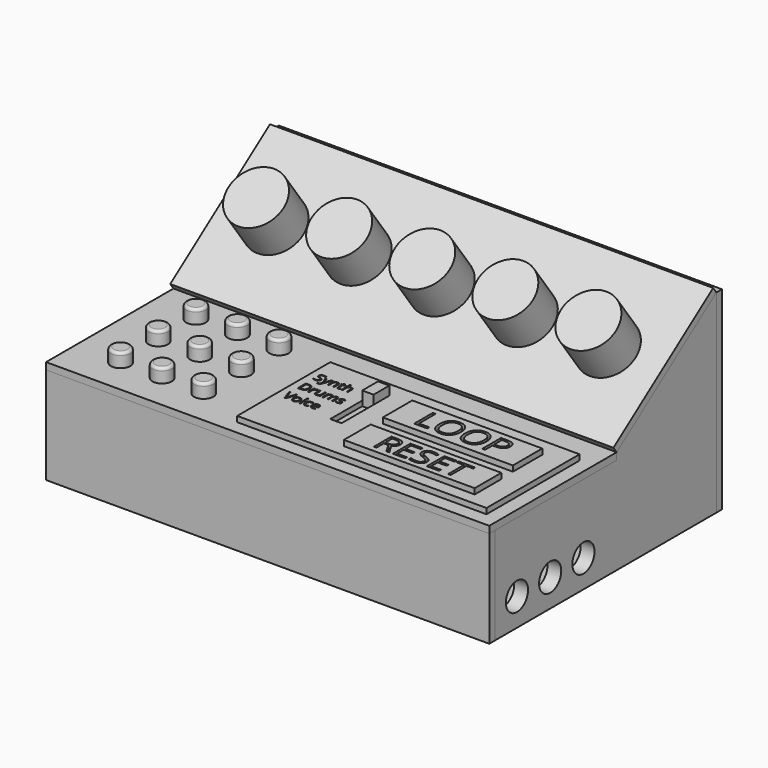
from build123d import *

# Parameters (mm, degrees)
F0_W          = 203.2
F0_H          = 127
F1_DEPTH      = 6.35
F2_W          = 63.5
F2_H          = 38.1
F3_DEPTH      = 6.35
F5_DEPTH      = 6.35
F6_W          = 203.2
F6_H          = 70.496440513
F7_DEPTH      = 3.175
F9_DEPTH      = 3.175
F10_W         = 203.2
F10_H         = 44.45
F11_DEPTH     = 3.175
F12_W         = 203.2
F12_H         = 88.9
F13_DEPTH     = 3.175
F14_R         = 12.7
F15_DEPTH     = 19.05
F16_R         = 6.35
F17_DEPTH     = 25.4
F18_R         = 26.0740110677
F19_DEPTH     = 6.35
F20_R         = 6.34999
F21_W         = 114.3
F21_H         = 53.34
F22_DEPTH     = 2.54
F23_TEXT_SIZE = 6.4763732048
F24_DEPTH     = 1.27
F25_W         = 5.1960833371
F25_H         = 27.3660402745
F26_DEPTH     = 2.286
F27_W         = 5.1960833371
F27_H         = 9.0065440163
F28_DEPTH     = 6.35
F29_W         = 59.6115607768
F29_H         = 16.8355405331
F30_DEPTH     = 2.54
F29_W_2       = 59.9551443011
F29_H_2       = 15.2894221246
F32_R         = 4.445
F33_DEPTH     = 6.35
F34_R         = 1.27
F34_2_R       = 1.27
F34_3_R       = 1.27
F34_4_R       = 1.27
F34_5_R       = 1.27
F34_6_R       = 1.27
F34_7_R       = 1.27
F34_8_R       = 1.27
F34_9_R       = 1.27


# Not quite as in the source:
# - a fillet or chamfer is up to 0.001 mm smaller than in the source, because OpenCascade refuses the exact size
# - Text() gives the source's letters only with a copy of the font that has no kerning and outlines rounded to 1/6400 em; it was checked with that copy


with BuildPart() as f1:
    # F0 (on Top) → F1 (new body)
    with BuildSketch(Plane.XY):
        Rectangle(F0_W, F0_H)
    extrude(amount=F1_DEPTH)

    # F2 (on face) → F3 (join)
    with BuildSketch(Plane(origin=(-101.6, 0, 0), x_dir=(0, -1, 0), z_dir=(-1, 0, 0))):
        Polygon((-63.5, 88.9), (-63.5, 6.35), (0, 6.35), (0, 44.45), (-6.35, 44.45), (-6.35, 47.625), align=None)
        with Locations((31.75, 25.4)):
            Rectangle(F2_W, F2_H)
    extrude(amount=-F3_DEPTH)

    # F4 (on face) → F5 (join)
    with BuildSketch(Plane.YZ.offset(101.6)):
        Polygon((-63.5, 44.45), (-63.5, 6.35), (63.5, 6.35), (63.5, 88.9), (6.35, 47.625), (6.35, 44.45), align=None)
    extrude(amount=-F5_DEPTH)

    # F16 (on face) → F17 (cut)
    with BuildSketch(Plane.YZ.offset(101.6)):
        with Locations((-50.8, 12.7)):
            Circle(F16_R)
        with Locations((-31.75, 12.7)):
            Circle(F16_R)
        with Locations((-12.7, 12.7)):
            Circle(F16_R)
    extrude(amount=-F17_DEPTH, mode=Mode.SUBTRACT)


with BuildPart() as f7:
    # F6 (on face) → F7 (new body)
    with BuildSketch(Plane(origin=(0, -20.4281947262, 28.2851926978), x_dir=(1, 0, 0), z_dir=(0, -0.5854905538, 0.8106792284))):
        with Locations((0, 68.2800209837)):
            Rectangle(F6_W, F6_H)
    extrude(amount=F7_DEPTH)


with BuildPart() as f9:
    # F8 (on face) → F9 (new body)
    with BuildSketch(Plane.XY.offset(44.45)):
        Polygon((101.6, 6.35), (-101.6, 6.35), (-101.6, -66.675), (101.6, -66.675), (101.6, -63.5), align=None)
    extrude(amount=F9_DEPTH)

    # F21 (on face) → F22 (join)
    with BuildSketch(Plane.XY.offset(47.625)):
        with Locations((38.1, -33.655)):
            Rectangle(F21_W, F21_H)
    extrude(amount=F22_DEPTH)

    # F23 (on face) → F24 (cut)
    with BuildSketch(Plane.XY.offset(50.165)):
        with Locations((-16.209024936, -21.1453055963)):
            Text('Synth', F23_TEXT_SIZE, font='Open Sans', text_align=(TextAlign.LEFT, TextAlign.BOTTOM))
        with Locations((-16.209024936, -29.9531731548)):
            Text('Drums', F23_TEXT_SIZE, font='Open Sans', text_align=(TextAlign.LEFT, TextAlign.BOTTOM))
        with Locations((-16.209024936, -38.7610407132)):
            Text('Voice', F23_TEXT_SIZE, font='Open Sans', text_align=(TextAlign.LEFT, TextAlign.BOTTOM))
    extrude(amount=-F24_DEPTH, mode=Mode.SUBTRACT)

    # F25 (on face) → F26 (cut)
    with BuildSketch(Plane.XY.offset(50.165)):
        with Locations((11.0760945827, -27.7290083468)):
            Rectangle(F25_W, F25_H)
    extrude(amount=-F26_DEPTH, mode=Mode.SUBTRACT)


with BuildPart() as f11:
    # F10 (on face) → F11 (new body)
    with BuildSketch(Plane.XZ.offset(63.5)):
        with Locations((0, 22.225)):
            Rectangle(F10_W, F10_H)
    extrude(amount=F11_DEPTH)


with BuildPart() as f13:
    # F12 (on face) → F13 (new body)
    with BuildSketch(Plane(origin=(0, 63.5, 0), x_dir=(-1, 0, 0), z_dir=(0, 1, 0))):
        with Locations((0, 44.45)):
            Rectangle(F12_W, F12_H)
    extrude(amount=F13_DEPTH)


with BuildPart() as f15:
    # F14 (on face) → F15 (new body)
    with BuildSketch(Plane(origin=(0, -22.2871272346, 30.8590992479), x_dir=(1, 0, 0), z_dir=(0, -0.5854905538, 0.8106792284))):
        with Locations((76.2, 68.2800209837)):
            Circle(F14_R)
    extrude(amount=F15_DEPTH)


with BuildPart() as f15b:
    # F14 (on face) → F15, piece 2 (new body)
    with BuildSketch(Plane(origin=(0, -22.2871272346, 30.8590992479), x_dir=(1, 0, 0), z_dir=(0, -0.5854905538, 0.8106792284))):
        with Locations((38.1, 68.2800209837)):
            Circle(F14_R)
    extrude(amount=F15_DEPTH)


with BuildPart() as f15c:
    # F14 (on face) → F15, piece 3 (new body)
    with BuildSketch(Plane(origin=(0, -22.2871272346, 30.8590992479), x_dir=(1, 0, 0), z_dir=(0, -0.5854905538, 0.8106792284))):
        with Locations((0, 68.2800209837)):
            Circle(F14_R)
    extrude(amount=F15_DEPTH)


with BuildPart() as f15d:
    # F14 (on face) → F15, piece 4 (new body)
    with BuildSketch(Plane(origin=(0, -22.2871272346, 30.8590992479), x_dir=(1, 0, 0), z_dir=(0, -0.5854905538, 0.8106792284))):
        with Locations((-38.1, 68.2800209837)):
            Circle(F14_R)
    extrude(amount=F15_DEPTH)


with BuildPart() as f15e:
    # F14 (on face) → F15, piece 5 (new body)
    with BuildSketch(Plane(origin=(0, -22.2871272346, 30.8590992479), x_dir=(1, 0, 0), z_dir=(0, -0.5854905538, 0.8106792284))):
        with Locations((-76.2, 68.2800209837)):
            Circle(F14_R)
    extrude(amount=F15_DEPTH)


with BuildPart() as f19:
    # F18 (on face) → F19 (new body)
    with BuildSketch(Plane.XY.offset(47.625)):
        with Locations((-63.5, -34.925)):
            Circle(F18_R)
    extrude(amount=F19_DEPTH)

    # F20 (radius 6.35 in the source; OpenCascade refuses exactly that, so slightly less here)
    f20_edges = [f19.edges().sort_by_distance(p)[0] for p in [
        (-89.574011, -34.925, 53.975),
    ]]
    fillet(f20_edges, radius=F20_R)


with BuildPart() as f28:
    # F27 (on face) → F28 (new body)
    with BuildSketch(Plane.XY.offset(47.879)):
        with Locations((11.0760945827, -18.5492602177)):
            Rectangle(F27_W, F27_H)
    extrude(amount=F28_DEPTH)


with BuildPart() as f30:
    # F29 (on face) → F30 (new body)
    with BuildSketch(Plane.XY.offset(50.165)):
        with Locations((55.256693624, -24.043854326)):
            Rectangle(F29_W, F29_H)
        Polygon((43.2155371847, -29.1975922883), (37.2333763145, -29.1975922883), (37.2333763145, -18.4663425765), (38.4805405948, -18.4663425765), (38.4805405948, -28.0678634392), (43.2155371847, -28.0678634392), align=None, mode=Mode.SUBTRACT)
        with BuildLine():
            add(Edge.make_bspline(
                [(53.05192891, -19.7651784466), (54.3507647801, -21.2331213378), (54.3507647801, -23.8167008263)],
                knots=[0, 0, 0, 1, 1, 1], degree=2))
            add(Edge.make_bspline(
                [(54.3507647801, -23.8167008263), (54.3507647801, -26.3932341889), (53.0472314927, -27.8693975603)],
                knots=[0, 0, 0, 1, 1, 1], degree=2))
            add(Edge.make_bspline(
                [(53.0472314927, -27.8693975603), (51.7436982053, -29.3455609317), (49.4255227916, -29.3455609317)],
                knots=[0, 0, 0, 1, 1, 1], degree=2))
            add(Edge.make_bspline(
                [(49.4255227916, -29.3455609317), (47.055675788, -29.3455609317), (45.7674091067, -27.8952333552)],
                knots=[0, 0, 0, 1, 1, 1], degree=2))
            add(Edge.make_bspline(
                [(45.7674091067, -27.8952333552), (44.4791424254, -26.4449057787), (44.4791424254, -23.8026085745)],
                knots=[0, 0, 0, 1, 1, 1], degree=2))
            add(Edge.make_bspline(
                [(44.4791424254, -23.8026085745), (44.4791424254, -21.181449748), (45.7709321696, -19.7393426517)],
                knots=[0, 0, 0, 1, 1, 1], degree=2))
            add(Edge.make_bspline(
                [(45.7709321696, -19.7393426517), (47.0627219139, -18.2972355554), (49.4396150433, -18.2972355554)],
                knots=[0, 0, 0, 1, 1, 1], degree=2))
            add(Edge.make_bspline(
                [(49.4396150433, -18.2972355554), (51.7530930398, -18.2972355554), (53.05192891, -19.7651784466)],
                knots=[0, 0, 0, 1, 1, 1], degree=2))
        make_face(mode=Mode.SUBTRACT)
        with BuildLine():
            add(Edge.make_bspline(
                [(64.7578927015, -19.7651784466), (66.0567285716, -21.2331213378), (66.0567285716, -23.8167008263)],
                knots=[0, 0, 0, 1, 1, 1], degree=2))
            add(Edge.make_bspline(
                [(66.0567285716, -23.8167008263), (66.0567285716, -26.3932341889), (64.7531952842, -27.8693975603)],
                knots=[0, 0, 0, 1, 1, 1], degree=2))
            add(Edge.make_bspline(
                [(64.7531952842, -27.8693975603), (63.4496619969, -29.3455609317), (61.1314865831, -29.3455609317)],
                knots=[0, 0, 0, 1, 1, 1], degree=2))
            add(Edge.make_bspline(
                [(61.1314865831, -29.3455609317), (58.7616395795, -29.3455609317), (57.4733728982, -27.8952333552)],
                knots=[0, 0, 0, 1, 1, 1], degree=2))
            add(Edge.make_bspline(
                [(57.4733728982, -27.8952333552), (56.1851062169, -26.4449057787), (56.1851062169, -23.8026085745)],
                knots=[0, 0, 0, 1, 1, 1], degree=2))
            add(Edge.make_bspline(
                [(56.1851062169, -23.8026085745), (56.1851062169, -21.181449748), (57.4768959612, -19.7393426517)],
                knots=[0, 0, 0, 1, 1, 1], degree=2))
            add(Edge.make_bspline(
                [(57.4768959612, -19.7393426517), (58.7686857054, -18.2972355554), (61.1455788348, -18.2972355554)],
                knots=[0, 0, 0, 1, 1, 1], degree=2))
            add(Edge.make_bspline(
                [(61.1455788348, -18.2972355554), (63.4590568314, -18.2972355554), (64.7578927015, -19.7651784466)],
                knots=[0, 0, 0, 1, 1, 1], degree=2))
        make_face(mode=Mode.SUBTRACT)
        with BuildLine():
            add(Edge.make_bspline(
                [(71.2309336745, -18.4663425765), (75.251922842, -18.4663425765), (75.251922842, -21.5924737576)],
                knots=[0, 0, 0, 1, 1, 1], degree=2))
            add(Edge.make_bspline(
                [(75.251922842, -21.5924737576), (75.251922842, -23.2224775439), (74.1398093077, -24.0997202157)],
                knots=[0, 0, 0, 1, 1, 1], degree=2))
            add(Edge.make_bspline(
                [(74.1398093077, -24.0997202157), (73.0276957733, -24.9769628875), (70.9584834739, -24.9769628875)],
                knots=[0, 0, 0, 1, 1, 1], degree=2))
            Line((70.9584834739, -24.9769628875), (69.6948782331, -24.9769628875))
            Line((69.6948782331, -24.9769628875), (69.6948782331, -29.1975922883))
            Line((69.6948782331, -29.1975922883), (68.4477139528, -29.1975922883))
            Line((68.4477139528, -29.1975922883), (68.4477139528, -18.4663425765))
            Line((68.4477139528, -18.4663425765), (71.2309336745, -18.4663425765))
        make_face(mode=Mode.SUBTRACT)
    extrude(amount=F30_DEPTH)


with BuildPart() as f30b:
    # F29 (on face) → F30, piece 2 (new body)
    with BuildSketch(Plane.XY.offset(50.165)):
        with Locations((55.4284853861, -47.1497792751)):
            Rectangle(F29_W_2, F29_H_2)
        with BuildLine():
            Line((40.4061070812, -48.0384091174), (38.3077044907, -48.0384091174))
            Line((38.3077044907, -48.0384091174), (38.3077044907, -52.217617631))
            Line((38.3077044907, -52.217617631), (37.1397256903, -52.217617631))
            Line((37.1397256903, -52.217617631), (37.1397256903, -42.1677209476))
            Line((37.1397256903, -42.1677209476), (39.8958037258, -42.1677209476))
            add(Edge.make_bspline(
                [(39.8958037258, -42.1677209476), (41.7456533889, -42.1677209476), (42.6287861353, -42.8759868114)],
                knots=[0, 0, 0, 1, 1, 1], degree=2))
            add(Edge.make_bspline(
                [(42.6287861353, -42.8759868114), (43.5119188818, -43.5842526753), (43.5119188818, -45.0073831534)],
                knots=[0, 0, 0, 1, 1, 1], degree=2))
            add(Edge.make_bspline(
                [(43.5119188818, -45.0073831534), (43.5119188818, -47.0002057393), (41.4905017112, -47.7018728529)],
                knots=[0, 0, 0, 1, 1, 1], degree=2))
            Line((41.4905017112, -47.7018728529), (44.2201847456, -52.217617631))
            Line((44.2201847456, -52.217617631), (42.8388463527, -52.217617631))
            Line((42.8388463527, -52.217617631), (40.4061070812, -48.0384091174))
        make_face(mode=Mode.SUBTRACT)
        Polygon((51.4436167238, -51.1728155026), (51.4436167238, -52.217617631), (45.8412777322, -52.217617631), (45.8412777322, -42.1677209476), (51.4436167238, -42.1677209476), (51.4436167238, -43.2059243257), (47.0092565326, -43.2059243257), (47.0092565326, -46.443711132), (51.1752675456, -46.443711132), (51.1752675456, -47.4753157598), (47.0092565326, -47.4753157598), (47.0092565326, -51.1728155026), align=None, mode=Mode.SUBTRACT)
        with BuildLine():
            add(Edge.make_bspline(
                [(58.7462337054, -47.86684161), (59.340121231, -48.5135191379), (59.340121231, -49.5429241823)],
                knots=[0, 0, 0, 1, 1, 1], degree=2))
            add(Edge.make_bspline(
                [(59.340121231, -49.5429241823), (59.340121231, -50.8692729895), (58.3778034812, -51.6127321882)],
                knots=[0, 0, 0, 1, 1, 1], degree=2))
            add(Edge.make_bspline(
                [(58.3778034812, -51.6127321882), (57.4154857313, -52.3561913869), (55.7657981602, -52.3561913869)],
                knots=[0, 0, 0, 1, 1, 1], degree=2))
            add(Edge.make_bspline(
                [(55.7657981602, -52.3561913869), (53.9797364165, -52.3561913869), (53.016318875, -51.894278867)],
                knots=[0, 0, 0, 1, 1, 1], degree=2))
            Line((53.016318875, -51.894278867), (53.016318875, -50.7680921518))
            add(Edge.make_bspline(
                [(53.016318875, -50.7680921518), (53.6366014017, -51.0276429963), (54.3646635164, -51.1794142529)],
                knots=[0, 0, 0, 1, 1, 1], degree=2))
            add(Edge.make_bspline(
                [(54.3646635164, -51.1794142529), (55.0927256312, -51.3311855094), (55.8075902453, -51.3311855094)],
                knots=[0, 0, 0, 1, 1, 1], degree=2))
            add(Edge.make_bspline(
                [(55.8075902453, -51.3311855094), (56.9755690457, -51.3311855094), (57.5672569879, -50.8879694486)],
                knots=[0, 0, 0, 1, 1, 1], degree=2))
            add(Edge.make_bspline(
                [(57.5672569879, -50.8879694486), (58.1589449301, -50.4447533878), (58.1589449301, -49.6529033537)],
                knots=[0, 0, 0, 1, 1, 1], degree=2))
            add(Edge.make_bspline(
                [(58.1589449301, -49.6529033537), (58.1589449301, -49.1316020812), (57.9488847127, -48.7983651918)],
                knots=[0, 0, 0, 1, 1, 1], degree=2))
            add(Edge.make_bspline(
                [(57.9488847127, -48.7983651918), (57.7388244953, -48.4651283025), (57.2472175991, -48.1824818319)],
                knots=[0, 0, 0, 1, 1, 1], degree=2))
            add(Edge.make_bspline(
                [(57.2472175991, -48.1824818319), (56.7556107029, -47.8998353614), (55.7526006596, -47.5435028461)],
                knots=[0, 0, 0, 1, 1, 1], degree=2))
            add(Edge.make_bspline(
                [(55.7526006596, -47.5435028461), (54.3514660159, -47.0419978244), (53.7498799483, -46.3546280031)],
                knots=[0, 0, 0, 1, 1, 1], degree=2))
            add(Edge.make_bspline(
                [(53.7498799483, -46.3546280031), (53.1482938806, -45.6672581818), (53.1482938806, -44.5608677174)],
                knots=[0, 0, 0, 1, 1, 1], degree=2))
            add(Edge.make_bspline(
                [(53.1482938806, -44.5608677174), (53.1482938806, -43.3994876674), (54.0204287099, -42.712117846)],
                knots=[0, 0, 0, 1, 1, 1], degree=2))
            add(Edge.make_bspline(
                [(54.0204287099, -42.712117846), (54.8925635392, -42.0247480247), (56.3310911012, -42.0247480247)],
                knots=[0, 0, 0, 1, 1, 1], degree=2))
            add(Edge.make_bspline(
                [(56.3310911012, -42.0247480247), (57.8290074158, -42.0247480247), (59.0871691367, -42.5746438818)],
                knots=[0, 0, 0, 1, 1, 1], degree=2))
            Line((59.0871691367, -42.5746438818), (58.7220382877, -43.5908514256))
            add(Edge.make_bspline(
                [(58.7220382877, -43.5908514256), (57.4770740673, -43.0695501531), (56.3024965167, -43.0695501531)],
                knots=[0, 0, 0, 1, 1, 1], degree=2))
            add(Edge.make_bspline(
                [(56.3024965167, -43.0695501531), (55.37427231, -43.0695501531), (54.8518712458, -43.4676747536)],
                knots=[0, 0, 0, 1, 1, 1], degree=2))
            add(Edge.make_bspline(
                [(54.8518712458, -43.4676747536), (54.3294701816, -43.8657993541), (54.3294701816, -44.574065218)],
                knots=[0, 0, 0, 1, 1, 1], degree=2))
            add(Edge.make_bspline(
                [(54.3294701816, -44.574065218), (54.3294701816, -45.0953664905), (54.5219337315, -45.4297031716)],
                knots=[0, 0, 0, 1, 1, 1], degree=2))
            add(Edge.make_bspline(
                [(54.5219337315, -45.4297031716), (54.7143972815, -45.7640398527), (55.1719106346, -46.0422871563)],
                knots=[0, 0, 0, 1, 1, 1], degree=2))
            add(Edge.make_bspline(
                [(55.1719106346, -46.0422871563), (55.6294239876, -46.32053446), (56.5708456949, -46.6570707245)],
                knots=[0, 0, 0, 1, 1, 1], degree=2))
            add(Edge.make_bspline(
                [(56.5708456949, -46.6570707245), (58.1523461798, -47.2201640821), (58.7462337054, -47.86684161)],
                knots=[0, 0, 0, 1, 1, 1], degree=2))
        make_face(mode=Mode.SUBTRACT)
        Polygon((66.9990707279, -51.1728155026), (66.9990707279, -52.217617631), (61.3967317363, -52.217617631), (61.3967317363, -42.1677209476), (66.9990707279, -42.1677209476), (66.9990707279, -43.2059243257), (62.5647105367, -43.2059243257), (62.5647105367, -46.443711132), (66.7307215497, -46.443711132), (66.7307215497, -47.4753157598), (62.5647105367, -47.4753157598), (62.5647105367, -51.1728155026), align=None, mode=Mode.SUBTRACT)
        Polygon((72.3176634573, -43.2059243257), (72.3176634573, -52.217617631), (71.1496846569, -52.217617631), (71.1496846569, -43.2059243257), (67.9668874363, -43.2059243257), (67.9668874363, -42.1677209476), (75.5004606779, -42.1677209476), (75.5004606779, -43.2059243257), align=None, mode=Mode.SUBTRACT)
    extrude(amount=F30_DEPTH)


with BuildPart() as f30c:
    # F29 (on face) → F30, piece 3 (new body)
    with BuildSketch(Plane.XY.offset(50.165)):
        with BuildLine():
            Line((69.6948782331, -19.5467485444), (69.6948782331, -23.9059517541))
            Line((69.6948782331, -23.9059517541), (70.819909665, -23.9059517541))
            add(Edge.make_bspline(
                [(70.819909665, -23.9059517541), (72.4780979548, -23.9059517541), (73.2191155263, -23.3704461874)],
                knots=[0, 0, 0, 1, 1, 1], degree=2))
            add(Edge.make_bspline(
                [(73.2191155263, -23.3704461874), (73.9601330978, -22.8349406207), (73.9601330978, -21.6511914732)],
                knots=[0, 0, 0, 1, 1, 1], degree=2))
            add(Edge.make_bspline(
                [(73.9601330978, -21.6511914732), (73.9601330978, -20.5872264657), (73.2625666359, -20.066987505)],
                knots=[0, 0, 0, 1, 1, 1], degree=2))
            add(Edge.make_bspline(
                [(73.2625666359, -20.066987505), (72.565000174, -19.5467485444), (71.0900111569, -19.5467485444)],
                knots=[0, 0, 0, 1, 1, 1], degree=2))
            Line((71.0900111569, -19.5467485444), (69.6948782331, -19.5467485444))
        make_face()
    extrude(amount=F30_DEPTH)


with BuildPart() as f30d:
    # F29 (on face) → F30, piece 4 (new body)
    with BuildSketch(Plane.XY.offset(50.165)):
        with BuildLine():
            add(Edge.make_bspline(
                [(58.4339947262, -20.5402522932), (57.5050804647, -21.6676324336), (57.5050804647, -23.8167008263)],
                knots=[0, 0, 0, 1, 1, 1], degree=2))
            add(Edge.make_bspline(
                [(57.5050804647, -23.8167008263), (57.5050804647, -25.9963024311), (58.4339947262, -27.1236825716)],
                knots=[0, 0, 0, 1, 1, 1], degree=2))
            add(Edge.make_bspline(
                [(58.4339947262, -27.1236825716), (59.3629089878, -28.251062712), (61.1314865831, -28.251062712)],
                knots=[0, 0, 0, 1, 1, 1], degree=2))
            add(Edge.make_bspline(
                [(61.1314865831, -28.251062712), (62.9141564301, -28.251062712), (63.8242810227, -27.1283799888)],
                knots=[0, 0, 0, 1, 1, 1], degree=2))
            add(Edge.make_bspline(
                [(63.8242810227, -27.1283799888), (64.7344056152, -26.0056972656), (64.7344056152, -23.8167008263)],
                knots=[0, 0, 0, 1, 1, 1], degree=2))
            add(Edge.make_bspline(
                [(64.7344056152, -23.8167008263), (64.7344056152, -21.6511914732), (63.8278040856, -20.532031813)],
                knots=[0, 0, 0, 1, 1, 1], degree=2))
            add(Edge.make_bspline(
                [(63.8278040856, -20.532031813), (62.921202556, -19.4128721527), (61.1455788348, -19.4128721527)],
                knots=[0, 0, 0, 1, 1, 1], degree=2))
            add(Edge.make_bspline(
                [(61.1455788348, -19.4128721527), (59.3629089878, -19.4128721527), (58.4339947262, -20.5402522932)],
                knots=[0, 0, 0, 1, 1, 1], degree=2))
        make_face()
    extrude(amount=F30_DEPTH)


with BuildPart() as f30e:
    # F29 (on face) → F30, piece 5 (new body)
    with BuildSketch(Plane.XY.offset(50.165)):
        with BuildLine():
            add(Edge.make_bspline(
                [(46.7280309347, -20.5402522932), (45.7991166732, -21.6676324336), (45.7991166732, -23.8167008263)],
                knots=[0, 0, 0, 1, 1, 1], degree=2))
            add(Edge.make_bspline(
                [(45.7991166732, -23.8167008263), (45.7991166732, -25.9963024311), (46.7280309347, -27.1236825716)],
                knots=[0, 0, 0, 1, 1, 1], degree=2))
            add(Edge.make_bspline(
                [(46.7280309347, -27.1236825716), (47.6569451962, -28.251062712), (49.4255227916, -28.251062712)],
                knots=[0, 0, 0, 1, 1, 1], degree=2))
            add(Edge.make_bspline(
                [(49.4255227916, -28.251062712), (51.2081926386, -28.251062712), (52.1183172312, -27.1283799888)],
                knots=[0, 0, 0, 1, 1, 1], degree=2))
            add(Edge.make_bspline(
                [(52.1183172312, -27.1283799888), (53.0284418237, -26.0056972656), (53.0284418237, -23.8167008263)],
                knots=[0, 0, 0, 1, 1, 1], degree=2))
            add(Edge.make_bspline(
                [(53.0284418237, -23.8167008263), (53.0284418237, -21.6511914732), (52.1218402941, -20.532031813)],
                knots=[0, 0, 0, 1, 1, 1], degree=2))
            add(Edge.make_bspline(
                [(52.1218402941, -20.532031813), (51.2152387645, -19.4128721527), (49.4396150433, -19.4128721527)],
                knots=[0, 0, 0, 1, 1, 1], degree=2))
            add(Edge.make_bspline(
                [(49.4396150433, -19.4128721527), (47.6569451962, -19.4128721527), (46.7280309347, -20.5402522932)],
                knots=[0, 0, 0, 1, 1, 1], degree=2))
        make_face()
    extrude(amount=F30_DEPTH)


with BuildPart() as f30f:
    # F29 (on face) → F30, piece 6 (new body)
    with BuildSketch(Plane.XY.offset(50.165)):
        with BuildLine():
            Line((38.3077044907, -43.1927268251), (38.3077044907, -47.0353990741))
            Line((38.3077044907, -47.0353990741), (39.9112008098, -47.0353990741))
            add(Edge.make_bspline(
                [(39.9112008098, -47.0353990741), (41.1473666965, -47.0353990741), (41.7247573464, -46.5437921779)],
                knots=[0, 0, 0, 1, 1, 1], degree=2))
            add(Edge.make_bspline(
                [(41.7247573464, -46.5437921779), (42.3021479962, -46.0521852817), (42.3021479962, -45.0689714893)],
                knots=[0, 0, 0, 1, 1, 1], degree=2))
            add(Edge.make_bspline(
                [(42.3021479962, -45.0689714893), (42.3021479962, -44.0725601964), (41.7148592209, -43.6326435107)],
                knots=[0, 0, 0, 1, 1, 1], degree=2))
            add(Edge.make_bspline(
                [(41.7148592209, -43.6326435107), (41.1275704456, -43.1927268251), (39.8276166395, -43.1927268251)],
                knots=[0, 0, 0, 1, 1, 1], degree=2))
            Line((39.8276166395, -43.1927268251), (38.3077044907, -43.1927268251))
        make_face()
    extrude(amount=F30_DEPTH)


with BuildPart() as f33:
    # F32 (on face) → F33 (new body)
    with BuildSketch(Plane.XY.offset(47.625)):
        with Locations((-61.5176196386, -7.0791699694)):
            Circle(F32_R)
    extrude(amount=F33_DEPTH)

    # F34#6
    f34_6_edges = [f33.edges().sort_by_distance(p)[0] for p in [
        (-65.96262, -7.07917, 53.975),
    ]]
    fillet(f34_6_edges, radius=F34_6_R)


with BuildPart() as f33b:
    # F32 (on face) → F33, piece 2 (new body)
    with BuildSketch(Plane.XY.offset(47.625)):
        with Locations((-42.4676196386, -7.0791699694)):
            Circle(F32_R)
    extrude(amount=F33_DEPTH)

    # F34#7
    f34_7_edges = [f33b.edges().sort_by_distance(p)[0] for p in [
        (-46.91262, -7.07917, 53.975),
    ]]
    fillet(f34_7_edges, radius=F34_7_R)


with BuildPart() as f33c:
    # F32 (on face) → F33, piece 3 (new body)
    with BuildSketch(Plane.XY.offset(47.625)):
        with Locations((-80.5676196386, -7.0791699694)):
            Circle(F32_R)
    extrude(amount=F33_DEPTH)

    # F34#5
    f34_5_edges = [f33c.edges().sort_by_distance(p)[0] for p in [
        (-85.01262, -7.07917, 53.975),
    ]]
    fillet(f34_5_edges, radius=F34_5_R)


with BuildPart() as f33d:
    # F32 (on face) → F33, piece 4 (new body)
    with BuildSketch(Plane.XY.offset(47.625)):
        with Locations((-80.5676196386, -28.6691699694)):
            Circle(F32_R)
    extrude(amount=F33_DEPTH)

    # F34
    f34_edges = [f33d.edges().sort_by_distance(p)[0] for p in [
        (-85.01262, -28.66917, 53.975),
    ]]
    fillet(f34_edges, radius=F34_R)


with BuildPart() as f33e:
    # F32 (on face) → F33, piece 5 (new body)
    with BuildSketch(Plane.XY.offset(47.625)):
        with Locations((-61.5176196386, -28.6691699694)):
            Circle(F32_R)
    extrude(amount=F33_DEPTH)

    # F34#4
    f34_4_edges = [f33e.edges().sort_by_distance(p)[0] for p in [
        (-65.96262, -28.66917, 53.975),
    ]]
    fillet(f34_4_edges, radius=F34_4_R)


with BuildPart() as f33f:
    # F32 (on face) → F33, piece 6 (new body)
    with BuildSketch(Plane.XY.offset(47.625)):
        with Locations((-42.4676196386, -28.6691699694)):
            Circle(F32_R)
    extrude(amount=F33_DEPTH)

    # F34#8
    f34_8_edges = [f33f.edges().sort_by_distance(p)[0] for p in [
        (-46.91262, -28.66917, 53.975),
    ]]
    fillet(f34_8_edges, radius=F34_8_R)


with BuildPart() as f33g:
    # F32 (on face) → F33, piece 7 (new body)
    with BuildSketch(Plane.XY.offset(47.625)):
        with Locations((-80.5676196386, -50.2591699694)):
            Circle(F32_R)
    extrude(amount=F33_DEPTH)

    # F34#2
    f34_2_edges = [f33g.edges().sort_by_distance(p)[0] for p in [
        (-85.01262, -50.25917, 53.975),
    ]]
    fillet(f34_2_edges, radius=F34_2_R)


with BuildPart() as f33h:
    # F32 (on face) → F33, piece 8 (new body)
    with BuildSketch(Plane.XY.offset(47.625)):
        with Locations((-61.5176196386, -50.2591699694)):
            Circle(F32_R)
    extrude(amount=F33_DEPTH)

    # F34#3
    f34_3_edges = [f33h.edges().sort_by_distance(p)[0] for p in [
        (-65.96262, -50.25917, 53.975),
    ]]
    fillet(f34_3_edges, radius=F34_3_R)


with BuildPart() as f33i:
    # F32 (on face) → F33, piece 9 (new body)
    with BuildSketch(Plane.XY.offset(47.625)):
        with Locations((-42.4676196386, -50.2591699694)):
            Circle(F32_R)
    extrude(amount=F33_DEPTH)

    # F34#9
    f34_9_edges = [f33i.edges().sort_by_distance(p)[0] for p in [
        (-46.91262, -50.25917, 53.975),
    ]]
    fillet(f34_9_edges, radius=F34_9_R)


solid = Compound([f1.part, f7.part, f9.part, f11.part, f13.part, f15.part, f15b.part, f15c.part, f15d.part, f15e.part, f28.part, f30.part, f30b.part, f30c.part, f30d.part, f30e.part, f30f.part, f33.part, f33b.part, f33c.part, f33d.part, f33e.part, f33f.part, f33g.part, f33h.part, f33i.part])
